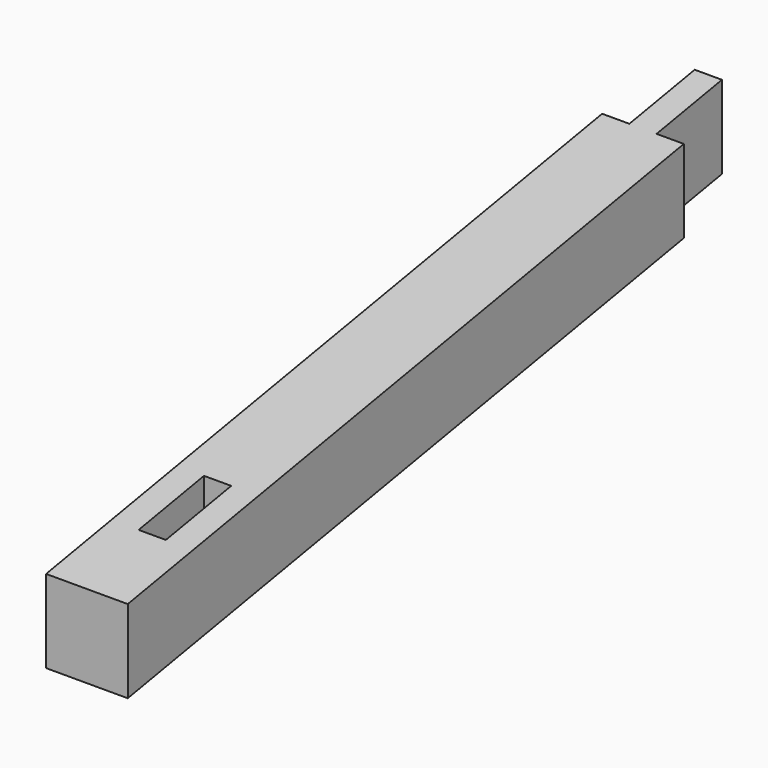
from build123d import *

# Parameters (mm, degrees)
F2_W      = 76.2
F2_H      = 749.3
F3_DEPTH  = 76.2
F5_W      = 25.4
F5_H      = 150.9289524655
F6_DEPTH  = 76.2
F7_W      = 88.9
F7_H      = 109.3234665417
F8_DEPTH  = 13.2329911382
F10_W     = 121.5671412647
F10_H     = 124.9910257757
F11_DEPTH = 25.4
F13_W     = 25.4
F13_H     = 183.5729926825
F14_DEPTH = 76.2


with BuildPart() as f3:
    # F2 (on face) → F3 (new body)
    with BuildSketch(Plane(origin=(0, -0.2741353876, 1.5546990396), x_dir=(1, 0, 0), z_dir=(0, -0.1736481777, 0.984807753))):
        with Locations((-23.2936060824, -27.5516035191)):
            Rectangle(F2_W, F2_H)
    extrude(amount=F3_DEPTH)

    # F5 (on face) → F6 (cut)
    with BuildSketch(Plane.XZ.offset(-328.3190653867)):
        with Locations((-48.6936060824, 61.4055776064)):
            Rectangle(F5_W, F5_H)
        with Locations((2.1063939176, 61.4055776064)):
            Rectangle(F5_W, F5_H)
    extrude(amount=F6_DEPTH, mode=Mode.SUBTRACT)

    # F7 (on face) → F8 (cut, through all)
    with BuildSketch(Plane.XZ.offset(-328.3190653867)):
        with Locations((-16.9436060824, 94.7153790316)):
            Rectangle(F7_W, F7_H)
    extrude(amount=-F8_DEPTH, mode=Mode.SUBTRACT)

    # F10 (on face) → F11 (cut)
    with BuildSketch(Plane(origin=(0, -396.3653928071, 0), x_dir=(-1, 0, 0), z_dir=(0, 1, 0))):
        with Locations((6.2730181962, -37.5579986721)):
            Rectangle(F10_W, F10_H)
    extrude(amount=-F11_DEPTH, mode=Mode.SUBTRACT)

    # F13 (on face) → F14 (cut)
    with BuildSketch(Plane(origin=(0, -243.9653928071, 0), x_dir=(-1, 0, 0), z_dir=(0, 1, 0))):
        with Locations((23.2936060824, -0.4609301686)):
            Rectangle(F13_W, F13_H)
    extrude(amount=-F14_DEPTH, mode=Mode.SUBTRACT)


solid = f3.part
